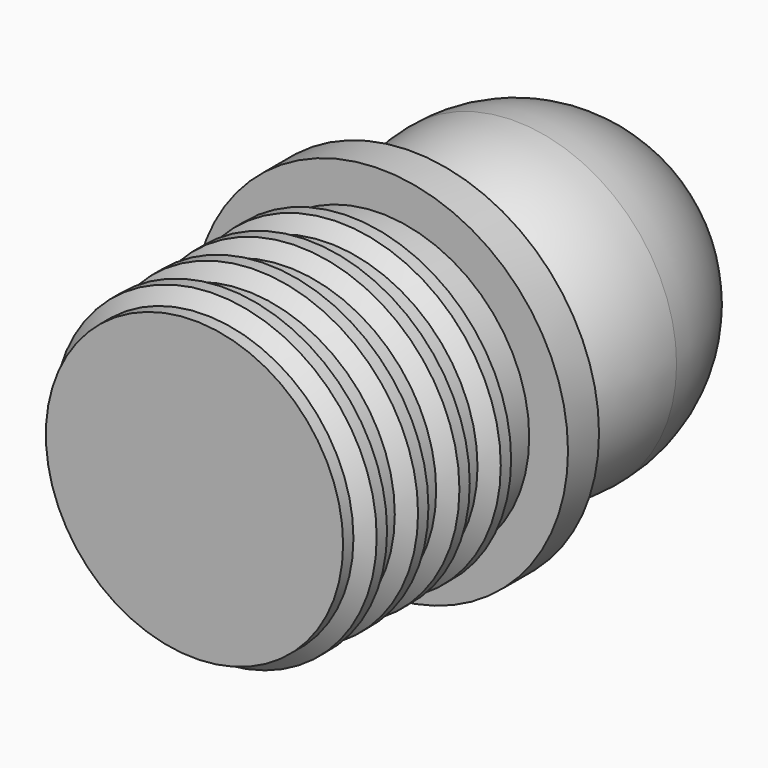
from build123d import *

# Parameters (mm, degrees)
F0_W    = 1
F0_H    = 1
F2_SIZE = 0.99999
F5_R    = 2


# Not quite as in the source:
# - a fillet or chamfer is up to 0.001 mm smaller than in the source, because OpenCascade refuses the exact size


with BuildPart() as f1:
    # F0 (on Top) → F1 (revolve)
    with BuildSketch(Plane.XY):
        Polygon((0, 21), (0, 0), (11.5, 0), (11.5, 2), (11.5, 3), (11.5, 6), (11.5, 7), (11.5, 10), (11.5, 11), (11.5, 14), (11.5, 15), (11.5, 18), (14.5, 18), (14.5, 21), align=None)
        with Locations((12, 14.5)):
            Rectangle(F0_W, F0_H)
        with Locations((12, 10.5)):
            Rectangle(F0_W, F0_H)
        with Locations((12, 6.5)):
            Rectangle(F0_W, F0_H)
        with Locations((12, 2.5)):
            Rectangle(F0_W, F0_H)
    revolve(axis=Axis((0, 10.5, 0), (0, 1, 0)))

    # F2 (size 1 in the source; OpenCascade refuses exactly that, so slightly less here)
    f2_edges = [f1.edges().sort_by_distance(p)[0] for p in [
        (-11.5, 2, 0),
        (-11.5, 6, 0),
        (-11.5, 10, 0),
        (-11.5, 14, 0),
    ]]
    chamfer(f2_edges, length=F2_SIZE)

    # F3 (on Top) → F4 (revolve)
    with BuildSketch(Plane.XY):
        with BuildLine():
            ThreePointArc((0, 18.5), (8.8388347648, 22.1611652352), (12.5, 31))
            ThreePointArc((12.5, 31), (8.8388347648, 39.8388347648), (0, 43.5))
            Line((0, 43.5), (0, 18.5))
        make_face()
    revolve(axis=Axis((0, 31, 0), (0, -1, 0)))

    # F5
    f5_edges = [f1.edges().sort_by_distance(p)[0] for p in [
        (-7.5, 21, 0),
    ]]
    fillet(f5_edges, radius=F5_R)


solid = f1.part
